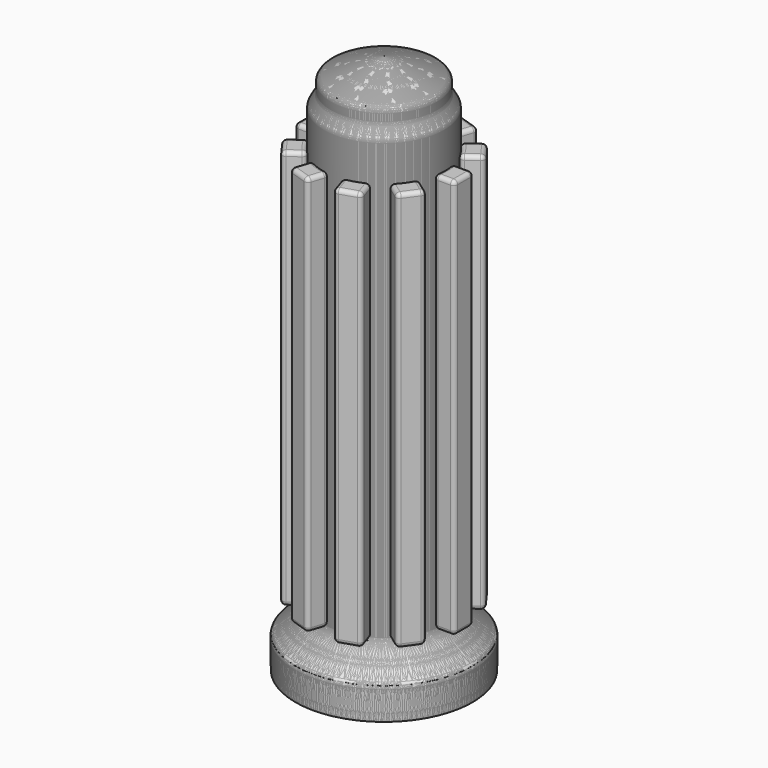
from build123d import *

# Parameters (mm, degrees)
F2_R     = 1.6
F4_W     = 6
F4_H     = 100
F6_R     = 1
F7_COUNT = 10


with BuildPart() as f1:
    # F0 (on Front) → F1 (revolve)
    with BuildSketch(Plane.XZ):
        with BuildLine():
            ThreePointArc((13.2958506606, 130.3251318397), (6.7693670842, 133.0079599221), (0, 135))
            Line((0, 135), (0, 125))
            Line((0, 125), (10.75, 125))
            Line((10.75, 125), (10.75, 0))
            Line((10.75, 0), (22.0892131329, 0))
            Line((22.0892131329, 0), (22.208115146, 8))
            Line((22.208115146, 8), (15, 14.0483267605))
            Line((15, 14.0483267605), (15, 124.0483267605))
            Line((15, 124.0483267605), (13.2958506606, 127))
            Line((13.2958506606, 127), (13.2958506606, 130.3251318397))
        make_face()
    revolve(axis=Axis((0, 0, 35.4471988976), (0, 0, 1)))

    # F2
    f2_edges = [f1.edges().sort_by_distance(p)[0] for p in [
        (-15, 0, 124.048327),
        (-13.295851, 0, 127),
        (-13.295851, 0, 130.325132),
        (6.769367, 0, 133.00796),
        (-15, 0, 14.048327),
        (-22.208115, 0, 8),
    ]]
    fillet(f2_edges, radius=F2_R)


with BuildPart() as f5:
    # F4 (on offset) → F5 (new body, up to the next surface of F1)
    with BuildSketch(Plane.YZ.offset(20)):
        with Locations((0, 65)):
            Rectangle(F4_W, F4_H)
    extrude(until=Until.NEXT, target=f1.part, dir=(-1, 0, 0))

    # F6
    f6_edges = [f5.edges().sort_by_distance(p)[0] for p in [
        (14.696938, -3, 65),
        (20, 3, 65),
        (20, -3, 65),
        (20, 0, 115),
        (17.348469, 3, 115),
        (14.924042, -1.507634, 115),
        (14.924042, 1.507634, 115),
        (17.348469, -3, 15),
        (20, 0, 15),
        (17.348469, -3, 115),
        (17.348469, 3, 15),
        (14.696938, 3, 65),
        (14.924042, 1.507634, 15),
        (14.924042, -1.507634, 15),
    ]]
    fillet(f6_edges, radius=F6_R)


with BuildPart() as f7_1:
    # F7: instance of F1
    add(f1.part.rotate(Axis((0, 0, 14.0483267605), (0, 0, 1)), 1 * 360 / F7_COUNT))


with BuildPart() as f7_2:
    # F7: instance of F1
    add(f1.part.rotate(Axis((0, 0, 14.0483267605), (0, 0, 1)), 2 * 360 / F7_COUNT))


with BuildPart() as f7_3:
    # F7: instance of F1
    add(f1.part.rotate(Axis((0, 0, 14.0483267605), (0, 0, 1)), 3 * 360 / F7_COUNT))


with BuildPart() as f7_4:
    # F7: instance of F1
    add(f1.part.rotate(Axis((0, 0, 14.0483267605), (0, 0, 1)), 4 * 360 / F7_COUNT))


with BuildPart() as f7_5:
    # F7: instance of F1
    add(f1.part.rotate(Axis((0, 0, 14.0483267605), (0, 0, 1)), 5 * 360 / F7_COUNT))


with BuildPart() as f7_6:
    # F7: instance of F1
    add(f1.part.rotate(Axis((0, 0, 14.0483267605), (0, 0, 1)), 6 * 360 / F7_COUNT))


with BuildPart() as f7_7:
    # F7: instance of F1
    add(f1.part.rotate(Axis((0, 0, 14.0483267605), (0, 0, 1)), 7 * 360 / F7_COUNT))


with BuildPart() as f7_8:
    # F7: instance of F1
    add(f1.part.rotate(Axis((0, 0, 14.0483267605), (0, 0, 1)), 8 * 360 / F7_COUNT))


with BuildPart() as f7_9:
    # F7: instance of F1
    add(f1.part.rotate(Axis((0, 0, 14.0483267605), (0, 0, 1)), 9 * 360 / F7_COUNT))


with BuildPart() as f7_10:
    # F7: instance of F5
    add(f5.part.rotate(Axis((0, 0, 14.0483267605), (0, 0, 1)), 1 * 360 / F7_COUNT))


with BuildPart() as f7_11:
    # F7: instance of F5
    add(f5.part.rotate(Axis((0, 0, 14.0483267605), (0, 0, 1)), 2 * 360 / F7_COUNT))


with BuildPart() as f7_12:
    # F7: instance of F5
    add(f5.part.rotate(Axis((0, 0, 14.0483267605), (0, 0, 1)), 3 * 360 / F7_COUNT))


with BuildPart() as f7_13:
    # F7: instance of F5
    add(f5.part.rotate(Axis((0, 0, 14.0483267605), (0, 0, 1)), 4 * 360 / F7_COUNT))


with BuildPart() as f7_14:
    # F7: instance of F5
    add(f5.part.rotate(Axis((0, 0, 14.0483267605), (0, 0, 1)), 5 * 360 / F7_COUNT))


with BuildPart() as f7_15:
    # F7: instance of F5
    add(f5.part.rotate(Axis((0, 0, 14.0483267605), (0, 0, 1)), 6 * 360 / F7_COUNT))


with BuildPart() as f7_16:
    # F7: instance of F5
    add(f5.part.rotate(Axis((0, 0, 14.0483267605), (0, 0, 1)), 7 * 360 / F7_COUNT))


with BuildPart() as f7_17:
    # F7: instance of F5
    add(f5.part.rotate(Axis((0, 0, 14.0483267605), (0, 0, 1)), 8 * 360 / F7_COUNT))


with BuildPart() as f7_18:
    # F7: instance of F5
    add(f5.part.rotate(Axis((0, 0, 14.0483267605), (0, 0, 1)), 9 * 360 / F7_COUNT))


solid = Compound([f1.part, f5.part, f7_1.part, f7_2.part, f7_3.part, f7_4.part, f7_5.part, f7_6.part, f7_7.part, f7_8.part, f7_9.part, f7_10.part, f7_11.part, f7_12.part, f7_13.part, f7_14.part, f7_15.part, f7_16.part, f7_17.part, f7_18.part])
